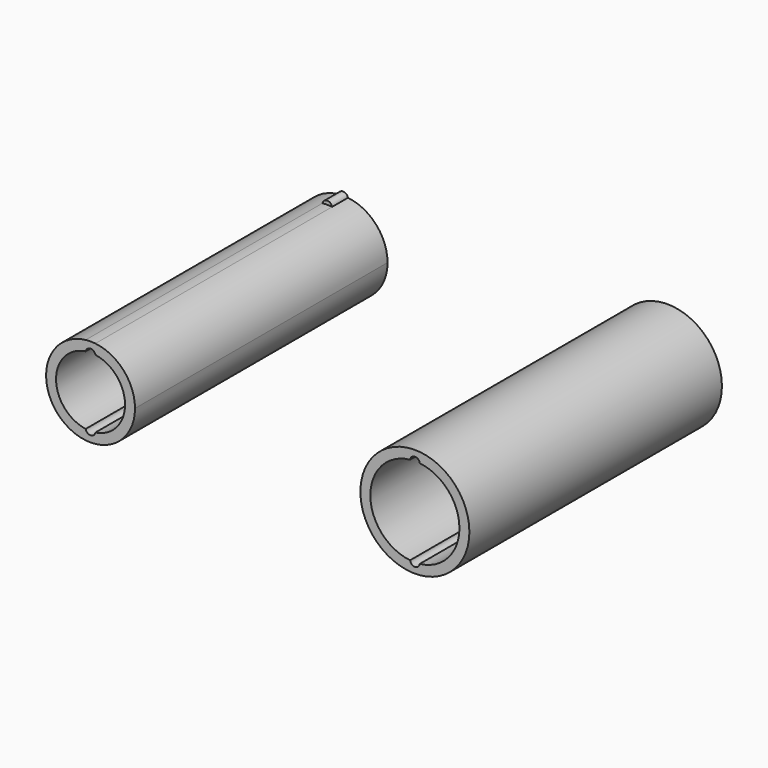
from build123d import *

# Parameters (mm, degrees)
F1_DEPTH = 50.8
F2_DEPTH = 3.175
F3_R     = 8.7691254342
F4_DEPTH = 50.8
F5_DEPTH = 1.5748


# Not quite as in the source:
# - a length typed as a fraction of an inch, garbled in the dataset ("3 / 203.2 mm" for 3/8 in), is restored
# - a feature names something its author has since deleted; it is built from what else it names


with BuildPart() as f1:
    # F0 (on Front) → F1 (new body)
    with BuildSketch(Plane.XZ):
        with BuildLine():
            ThreePointArc((-51.4129851972, -7.1128706299), (-46.8661970111, -4.7751922682), (-45.0398449824, 0))
            ThreePointArc((-45.0398449824, 0), (-46.8661970111, 4.7751922682), (-51.4129851972, 7.1128706299))
            ThreePointArc((-51.4129851972, 7.1128706299), (-52.1956458688, 7.1558008863), (-52.9783065404, 7.1128706299))
            ThreePointArc((-52.9783065404, 7.1128706299), (-59.3514467551, 0), (-52.9783065404, -7.1128706299))
            ThreePointArc((-52.9783065404, -7.1128706299), (-52.1956458688, -7.1558008863), (-51.4129851972, -7.1128706299))
        make_face()
        with BuildLine():
            ThreePointArc((-51.4129851972, 5.4954455624), (-48.0029766717, 3.6378571523), (-46.6447468735, 0))
            ThreePointArc((-46.6447468735, 0), (-48.0029766717, -3.6378571523), (-51.4129851972, -5.4954455624))
            ThreePointArc((-51.4129851972, -5.4954455624), (-52.1956458688, -6.1481072421), (-52.9783065404, -5.4954455624))
            ThreePointArc((-52.9783065404, -5.4954455624), (-57.7465448641, 0), (-52.9783065404, 5.4954455624))
            ThreePointArc((-52.9783065404, 5.4954455624), (-52.1956458688, 6.1481072421), (-51.4129851972, 5.4954455624))
        make_face(mode=Mode.SUBTRACT)
    extrude(amount=F1_DEPTH)

    # F0 (on Front) → F2 (join)
    with BuildSketch(Plane.XZ):
        with BuildLine():
            ThreePointArc((-51.4129851972, -7.1128706299), (-46.8661970111, -4.7751922682), (-45.0398449824, 0))
            ThreePointArc((-45.0398449824, 0), (-46.8661970111, 4.7751922682), (-51.4129851972, 7.1128706299))
            ThreePointArc((-51.4129851972, 7.1128706299), (-52.1956458688, 7.1558008863), (-52.9783065404, 7.1128706299))
            ThreePointArc((-52.9783065404, 7.1128706299), (-59.3514467551, 0), (-52.9783065404, -7.1128706299))
            ThreePointArc((-52.9783065404, -7.1128706299), (-52.1956458688, -7.1558008863), (-51.4129851972, -7.1128706299))
        make_face()
        with BuildLine():
            ThreePointArc((-51.4129851972, 5.4954455624), (-48.0029766717, 3.6378571523), (-46.6447468735, 0))
            ThreePointArc((-46.6447468735, 0), (-48.0029766717, -3.6378571523), (-51.4129851972, -5.4954455624))
            ThreePointArc((-51.4129851972, -5.4954455624), (-52.1956458688, -6.1481072421), (-52.9783065404, -5.4954455624))
            ThreePointArc((-52.9783065404, -5.4954455624), (-57.7465448641, 0), (-52.9783065404, 5.4954455624))
            ThreePointArc((-52.9783065404, 5.4954455624), (-52.1956458688, 6.1481072421), (-51.4129851972, 5.4954455624))
        make_face(mode=Mode.SUBTRACT)
        with BuildLine():
            ThreePointArc((-52.9783065404, 5.4954455624), (-52.1956458688, 5.5508989953), (-51.4129851972, 5.4954455624))
            ThreePointArc((-51.4129851972, 5.4954455624), (-52.1956458688, 6.1481072421), (-52.9783065404, 5.4954455624))
        make_face()
        with BuildLine():
            ThreePointArc((-52.9783065404, -5.4954455624), (-52.1956458688, -6.1481072421), (-51.4129851972, -5.4954455624))
            ThreePointArc((-51.4129851972, -5.4954455624), (-52.1956458688, -5.5508989953), (-52.9783065404, -5.4954455624))
        make_face()
        with BuildLine():
            ThreePointArc((-52.9783065404, 7.1128706299), (-52.1956458688, 7.1558008863), (-51.4129851972, 7.1128706299))
            ThreePointArc((-51.4129851972, 7.1128706299), (-52.1956458688, 7.7496697029), (-52.9783065404, 7.1128706299))
        make_face()
        with BuildLine():
            ThreePointArc((-52.9783065404, -7.1128706299), (-52.1956458688, -7.7496697029), (-51.4129851972, -7.1128706299))
            ThreePointArc((-51.4129851972, -7.1128706299), (-52.1956458688, -7.1558008863), (-52.9783065404, -7.1128706299))
        make_face()
    extrude(amount=F2_DEPTH)


with BuildPart() as f4:
    # F3 (on Front) → F4 (new body)
    with BuildSketch(Plane.XZ):
        Circle(F3_R)
        with BuildLine():
            ThreePointArc((0.793711748, 7.1235415414), (5.3415283007, 4.779424426), (7.1676232066, 0))
            ThreePointArc((7.1676232066, 0), (5.3415283007, -4.779424426), (0.793711748, -7.1235415414))
            ThreePointArc((0.793711748, -7.1235415414), (0.0099196257, -7.8095114052), (-0.7756125997, -7.1255348941))
            ThreePointArc((-0.7756125997, -7.1255348941), (-7.1676232066, 0), (-0.7756125997, 7.1255348941))
            ThreePointArc((-0.7756125997, 7.1255348941), (0.0099196257, 7.8095114052), (0.793711748, 7.1235415414))
        make_face(mode=Mode.SUBTRACT)
    extrude(amount=F4_DEPTH)

    # F3 (on Front) → F5 (join)
    with BuildSketch(Plane.XZ):
        with BuildLine():
            ThreePointArc((-0.7756125997, 7.1255348941), (0.0091042933, 7.1676174244), (0.793711748, 7.1235415414))
            ThreePointArc((0.793711748, 7.1235415414), (0.0099196257, 7.8095114052), (-0.7756125997, 7.1255348941))
        make_face()
        with BuildLine():
            ThreePointArc((-0.7756125997, -7.1255348941), (0.0099196257, -7.8095114052), (0.793711748, -7.1235415414))
            ThreePointArc((0.793711748, -7.1235415414), (0.0091042933, -7.1676174244), (-0.7756125997, -7.1255348941))
        make_face()
    extrude(amount=F5_DEPTH)


solid = Compound([f1.part, f4.part])
